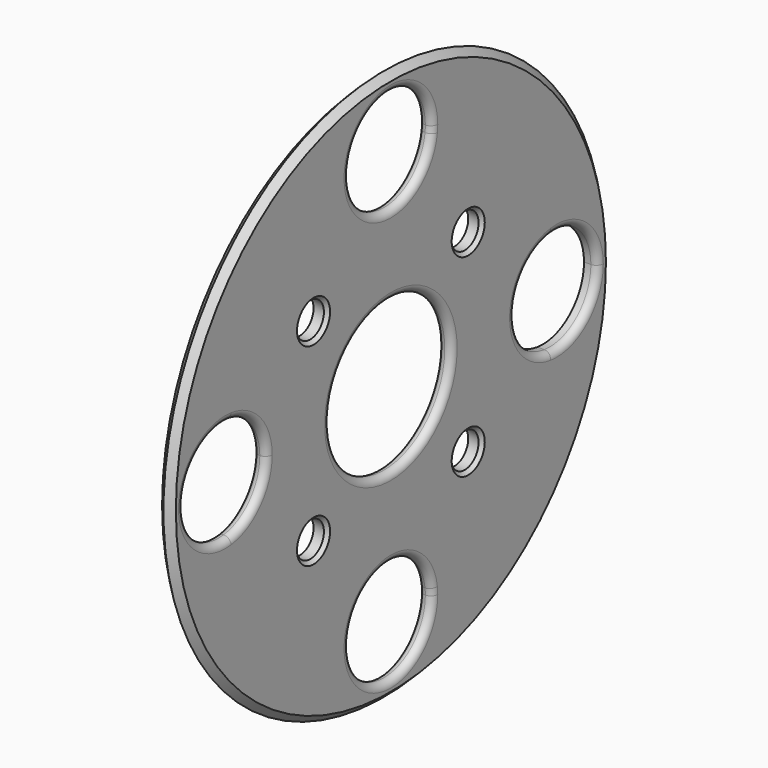
from build123d import *

# Parameters (mm, degrees)
F0_R     = 40
F0_R_2   = 2.5
F0_R_3   = 11.0176496963
F1_DEPTH = 2
F2_R     = 0.99999
F3_SIZE  = 0.99999
F4_SIZE  = 0.5
F5_R     = 0.99999


# Not quite as in the source:
# - a fillet or chamfer is up to 0.001 mm smaller than in the source, because OpenCascade refuses the exact size


with BuildPart() as f1:
    # F0 (on Right) → F1 (new body)
    with BuildSketch(Plane.YZ):
        Circle(F0_R)
        with BuildLine():
            ThreePointArc((7.4412717263, 29.0877185034), (21.2304956682, 21.2304956682), (29.0877185034, 7.4412717263))
            ThreePointArc((29.0877185034, 7.4412717263), (34.985527221, 5.6247454631), (37.5244549099, 0))
            ThreePointArc((37.5244549099, 0), (34.985527221, -5.6247454631), (29.0877185034, -7.4412717263))
            ThreePointArc((29.0877185034, -7.4412717263), (21.2304956682, -21.2304956682), (7.4412717263, -29.0877185034))
            ThreePointArc((7.4412717263, -29.0877185034), (7.4853035325, -29.5551671236), (7.5, -30.0244549099))
            ThreePointArc((7.5, -30.0244549099), (-0.4692877863, -37.5097584424), (-7.4412717263, -29.0877185034))
            ThreePointArc((-7.4412717263, -29.0877185034), (-21.2304956682, -21.2304956682), (-29.0877185034, -7.4412717263))
            ThreePointArc((-29.0877185034, -7.4412717263), (-37.5244549099, 0), (-29.0877185034, 7.4412717263))
            ThreePointArc((-29.0877185034, 7.4412717263), (-21.2304956682, 21.2304956682), (-7.4412717263, 29.0877185034))
            ThreePointArc((-7.4412717263, 29.0877185034), (-0.4692877863, 37.5097584424), (7.5, 30.0244549099))
            ThreePointArc((7.5, 30.0244549099), (7.4853035325, 29.5551671236), (7.4412717263, 29.0877185034))
        make_face(mode=Mode.SUBTRACT)
        with BuildLine():
            ThreePointArc((29.0877185034, -7.4412717263), (22.5244549099, 0), (29.0877185034, 7.4412717263))
            ThreePointArc((29.0877185034, 7.4412717263), (21.2304956682, 21.2304956682), (7.4412717263, 29.0877185034))
            ThreePointArc((7.4412717263, 29.0877185034), (0, 22.5244549099), (-7.4412717263, 29.0877185034))
            ThreePointArc((-7.4412717263, 29.0877185034), (-21.2304956682, 21.2304956682), (-29.0877185034, 7.4412717263))
            ThreePointArc((-29.0877185034, 7.4412717263), (-24.3997094468, 4.9610723111), (-22.5244549099, 0))
            ThreePointArc((-22.5244549099, 0), (-24.3997094468, -4.9610723111), (-29.0877185034, -7.4412717263))
            ThreePointArc((-29.0877185034, -7.4412717263), (-21.2304956682, -21.2304956682), (-7.4412717263, -29.0877185034))
            ThreePointArc((-7.4412717263, -29.0877185034), (0, -22.5244549099), (7.4412717263, -29.0877185034))
            ThreePointArc((7.4412717263, -29.0877185034), (21.2304956682, -21.2304956682), (29.0877185034, -7.4412717263))
        make_face()
        with Locations((-14.0257067978, -14.0257067978)):
            Circle(F0_R_2, mode=Mode.SUBTRACT)
        with Locations((14.0257067978, -14.0257067978)):
            Circle(F0_R_2, mode=Mode.SUBTRACT)
        with Locations((-14.0257067978, 14.0257067978)):
            Circle(F0_R_2, mode=Mode.SUBTRACT)
        Circle(F0_R_3, mode=Mode.SUBTRACT)
        with Locations((14.0257067978, 14.0257067978)):
            Circle(F0_R_2, mode=Mode.SUBTRACT)
    extrude(amount=F1_DEPTH)

    # F2 (radius 1 in the source; OpenCascade refuses exactly that, so slightly less here)
    f2_edges = [f1.edges().sort_by_distance(p)[0] for p in [
        (0, -11.01765, 0),
        (1, 11.01765, 0),
        (2, -11.01765, 0),
    ]]
    fillet(f2_edges, radius=F2_R)

    # F3 (size 1 in the source; OpenCascade refuses exactly that, so slightly less here)
    f3_edges = [f1.edges().sort_by_distance(p)[0] for p in [
        (0, -40, 0),
        (2, -40, 0),
    ]]
    chamfer(f3_edges, length=F3_SIZE)

    # F4
    f4_edges = [f1.edges().sort_by_distance(p)[0] for p in [
        (2, 11.525707, 14.025707),
        (2, 11.525707, -14.025707),
        (2, -16.525707, -14.025707),
        (2, -16.525707, 14.025707),
    ]]
    chamfer(f4_edges, length=F4_SIZE)

    # F5 (radius 1 in the source; OpenCascade refuses exactly that, so slightly less here)
    f5_edges = [f1.edges().sort_by_distance(p)[0] for p in [
        (2, -7.5, 30.024455),
        (2, 22.524455, 0),
        (2, -7.5, -30.024455),
        (2, -30.961191, -7.441272),
        (0, -30.961191, -7.441272),
        (0, -7.5, 30.024455),
        (0, -7.5, -30.024455),
    ]]
    fillet(f5_edges, radius=F5_R)


solid = f1.part
